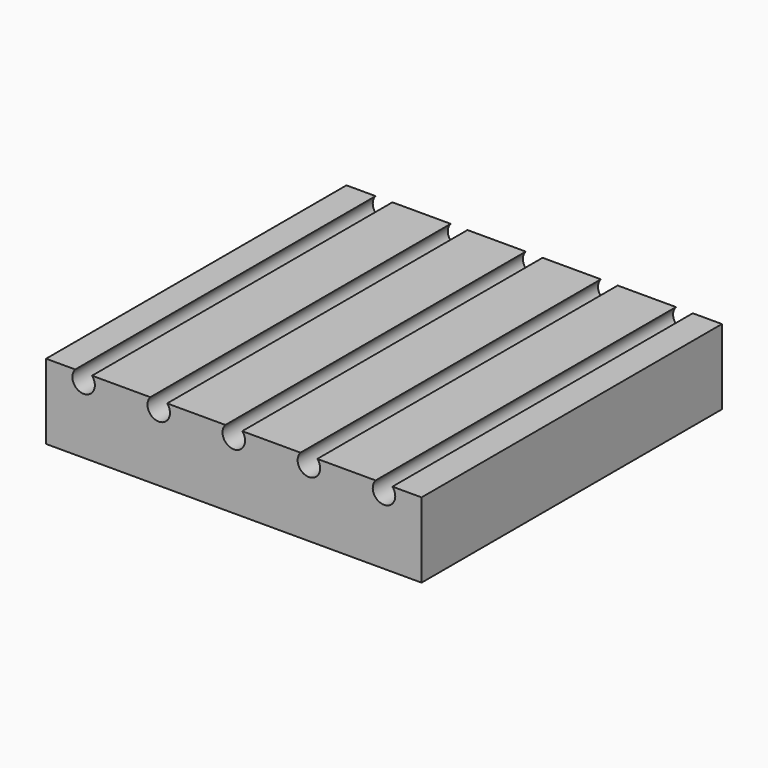
from build123d import *

# Parameters (mm, degrees)
F0_W     = 50
F0_H     = 50
F1_DEPTH = 10
F3_DEPTH = 50.001


# Not quite as in the source:
# - a feature names something its author has since deleted; it is built from what else it names


with BuildPart() as f1:
    # F0 (on Top) → F1 (new body)
    with BuildSketch(Plane.XY):
        Rectangle(F0_W, F0_H)
    extrude(amount=F1_DEPTH)

    # F2 (on face) → F3 (cut, through all)
    with BuildSketch(Plane.XZ.offset(25)):
        with BuildLine():
            Line((8.8819660113, 10), (11.1180339887, 10))
            ThreePointArc((11.1180339887, 10), (10, 10.5), (8.8819660113, 10))
        make_face()
        with BuildLine():
            ThreePointArc((1.1180339887, 10), (0, 10.5), (-1.1180339887, 10))
            Line((-1.1180339887, 10), (1.1180339887, 10))
        make_face()
        with BuildLine():
            ThreePointArc((-8.8819660113, 10), (-10, 10.5), (-11.1180339887, 10))
            Line((-11.1180339887, 10), (-8.8819660113, 10))
        make_face()
        with BuildLine():
            ThreePointArc((-18.8819660113, 10), (-20, 10.5), (-21.1180339887, 10))
            Line((-21.1180339887, 10), (-18.8819660113, 10))
        make_face()
        with BuildLine():
            ThreePointArc((11.5, 9), (11.4012585384, 9.5352331347), (11.1180339887, 10))
            Line((11.1180339887, 10), (8.8819660113, 10))
            ThreePointArc((8.8819660113, 10), (9.4647668653, 7.5987414616), (11.5, 9))
        make_face()
        with BuildLine():
            Line((1.1180339887, 10), (-1.1180339887, 10))
            ThreePointArc((-1.1180339887, 10), (-0.5352331347, 7.5987414616), (1.5, 9))
            ThreePointArc((1.5, 9), (1.4012585384, 9.5352331347), (1.1180339887, 10))
        make_face()
        with BuildLine():
            Line((-8.8819660113, 10), (-11.1180339887, 10))
            ThreePointArc((-11.1180339887, 10), (-10.5352331347, 7.5987414616), (-8.5, 9))
            ThreePointArc((-8.5, 9), (-8.5987414616, 9.5352331347), (-8.8819660113, 10))
        make_face()
        with BuildLine():
            Line((-18.8819660113, 10), (-21.1180339887, 10))
            ThreePointArc((-21.1180339887, 10), (-20.5352331347, 7.5987414616), (-18.5, 9))
            ThreePointArc((-18.5, 9), (-18.5987414616, 9.5352331347), (-18.8819660113, 10))
        make_face()
        with BuildLine():
            ThreePointArc((21.5, 9), (21.4012585384, 9.5352331347), (21.1180339887, 10))
            Line((21.1180339887, 10), (18.8819660113, 10))
            ThreePointArc((18.8819660113, 10), (19.4647668653, 7.5987414616), (21.5, 9))
        make_face()
    extrude(amount=-F3_DEPTH, mode=Mode.SUBTRACT)


solid = f1.part
